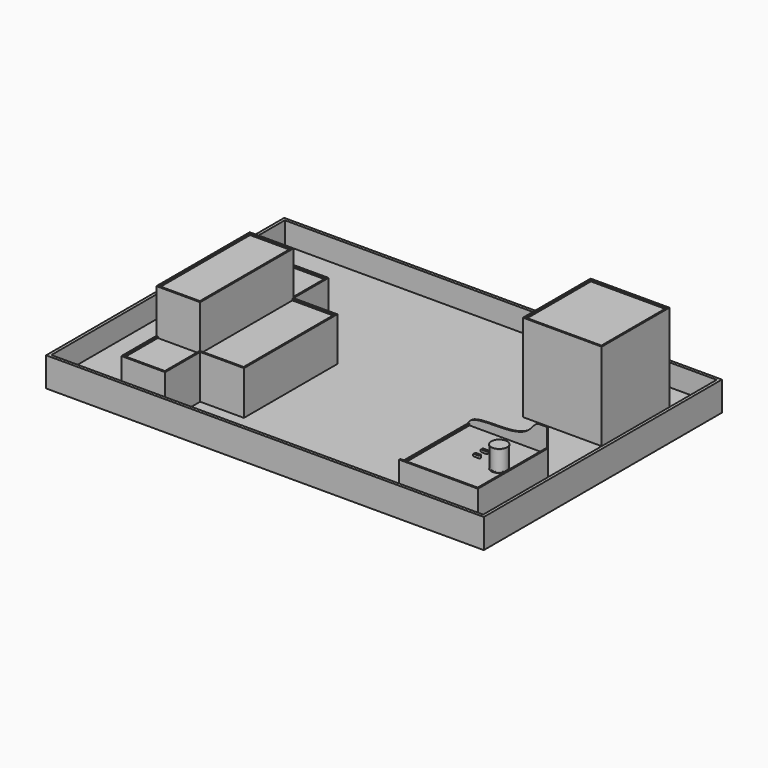
from build123d import *

# Parameters (mm, degrees)
F0_R      = 27.2
F1_DEPTH  = 2.83
F2_R      = 26.4
F3_DEPTH  = 67.36
F4_R      = 27.2
F5_DEPTH  = 2.83
F8_W      = 270
F8_H      = 300
F9_DEPTH  = 72
F11_DEPTH = 15
F13_DEPTH = 5
F14_W     = 5
F14_H     = 290
F15_DEPTH = 5
F16_W     = 1500
F16_H     = 1020
F17_DEPTH = 25
F18_W     = 270
F18_H     = 290
F19_DEPTH = 300
F20_W     = 260
F20_H     = 280
F21_DEPTH = 5
F22_W     = 1500
F22_H     = 1020
F22_W_2   = 1480
F22_H_2   = 1000
F23_DEPTH = 75
F25_DEPTH = 150
F26_W     = 150
F26_H     = 400
F27_DEPTH = 150
F28_W     = 140
F28_H     = 390
F29_DEPTH = 5
F30_W     = 140
F30_H     = 145
F30_W_2   = 145
F30_H_2   = 390
F31_DEPTH = 5
F32_R     = 3
F33_DEPTH = 4
F34_R     = 3.99999
F34_2_R   = 3.99999
F35_R     = 3
F36_DEPTH = 8
F37_R     = 3
F38_DEPTH = 8
F39_R     = 3
F39_R_2   = 2.5
F40_DEPTH = 3
F41_R     = 3
F41_R_2   = 2.5
F42_DEPTH = 3


# Not quite as in the source:
# - a fillet or chamfer is up to 0.001 mm smaller than in the source, because OpenCascade refuses the exact size
# - a feature names something its author has since deleted; it is built from what else it names


with BuildPart() as f1:
    # F0 (on Top) → F1 (new body)
    with BuildSketch(Plane.XY):
        Circle(F0_R)
    extrude(amount=F1_DEPTH)

    # F2 (on face) → F3 (join)
    with BuildSketch(Plane.XY.offset(2.83)):
        Circle(F2_R)
    extrude(amount=F3_DEPTH)

    # F4 (on face) → F5 (join)
    with BuildSketch(Plane.XY.offset(70.19)):
        Circle(F4_R)
    extrude(amount=F5_DEPTH)


with BuildPart() as f9:
    # F8 (on Top) → F9 (new body)
    with BuildSketch(Plane.XY):
        with Locations((-87.8, 0)):
            Rectangle(F8_W, F8_H)
    extrude(amount=-F9_DEPTH)

    # F10 (on face) → F11 (join)
    with BuildSketch(Plane.XY):
        Polygon((-222.8, -145), (-222.8, -150), (47.2, -150), (47.2, 150), (42.2, 150), (42.2, -145), align=None)
    extrude(amount=F11_DEPTH)

    # F12 (on face) → F13 (join)
    with BuildSketch(Plane(origin=(0, 150, 0), x_dir=(-1, 0, 0), z_dir=(0, 1, 0))):
        with BuildLine():
            Line((-21.3134280931, 81.3575685024), (-47.2, 81.3575685024))
            Line((-47.2, 81.3575685024), (-47.2, -72))
            Line((-47.2, -72), (222.8, -72))
            Line((222.8, -72), (222.8, 0))
            add(Edge.make_bspline(
                [(-21.3134280931, 81.3575685024), (-6.3059147253, 81.3822787863), (12.9585432644, 38.1268753575), (103.6097013063, 23.6068887567), (223.0224295336, 30.7718731823), (222.8, 0)],
                knots=[0, 0, 0, 0, 0.2487100673, 0.6151112321, 1, 1, 1, 1], degree=3))
        make_face()
    extrude(amount=-F13_DEPTH)

    # F14 (on face) → F15 (join)
    with BuildSketch(Plane.XY):
        with Locations((-220.3, 0)):
            Rectangle(F14_W, F14_H)
    extrude(amount=F15_DEPTH)

    # F16 (on face) → F17 (join)
    with BuildSketch(Plane(origin=(0, 0, -72), x_dir=(1, 0, 0), z_dir=(0, 0, -1))):
        with Locations((-602.8, -260)):
            Rectangle(F16_W, F16_H)
    extrude(amount=F17_DEPTH)

    # F18 (on face) → F19 (join)
    with BuildSketch(Plane.XY.offset(-72)):
        with Locations((-87.8, 525)):
            Rectangle(F18_W, F18_H)
    extrude(amount=F19_DEPTH)

    # F20 (on face) → F21 (cut)
    with BuildSketch(Plane.XY.offset(228)):
        with Locations((-87.8, 525)):
            Rectangle(F20_W, F20_H)
    extrude(amount=-F21_DEPTH, mode=Mode.SUBTRACT)

    # F22 (on face) → F23 (join)
    with BuildSketch(Plane.XY.offset(-72)):
        with Locations((-602.8, 260)):
            Rectangle(F22_W, F22_H)
        with Locations((-602.8, 260)):
            Rectangle(F22_W_2, F22_H_2, mode=Mode.SUBTRACT)
    extrude(amount=F23_DEPTH)

    # F24 (on face) → F25 (join)
    with BuildSketch(Plane.XY.offset(-72)):
        Polygon((-952.8, 460), (-1102.8, 460), (-1102.8, -240), (-952.8, -240), (-952.8, -90), (-802.8, -90), (-802.8, 310), (-952.8, 310), align=None)
    extrude(amount=F25_DEPTH)

    # F26 (on face) → F27 (join)
    with BuildSketch(Plane.XY.offset(78)):
        with Locations((-1027.8, 110)):
            Rectangle(F26_W, F26_H)
    extrude(amount=F27_DEPTH)

    # F28 (on face) → F29 (cut)
    with BuildSketch(Plane.XY.offset(228)):
        with Locations((-1027.8, 110)):
            Rectangle(F28_W, F28_H)
    extrude(amount=-F29_DEPTH, mode=Mode.SUBTRACT)

    # F30 (on face) → F31 (cut)
    with BuildSketch(Plane.XY.offset(78)):
        with Locations((-1027.8, 382.5)):
            Rectangle(F30_W, F30_H)
        with Locations((-880.3, 110)):
            Rectangle(F30_W_2, F30_H_2)
        with Locations((-1027.8, -162.5)):
            Rectangle(F30_W, F30_H)
    extrude(amount=-F31_DEPTH, mode=Mode.SUBTRACT)


with BuildPart() as f33:
    # F32 (on offset) → F33 (new body, symmetric)
    with BuildSketch(Plane.XY.offset(25)):
        with BuildLine():
            Line((-55, -12), (-74.5, -12))
            Line((-74.5, -12), (-74.5, -13))
            Line((-74.5, -13), (-65.6457513111, -13))
            ThreePointArc((-65.6457513111, -13), (-67, -16), (-65.6457513111, -19))
            Line((-65.6457513111, -19), (-74.5, -19))
            Line((-74.5, -19), (-74.5, -20))
            Line((-74.5, -20), (-55, -20))
            ThreePointArc((-55, -20), (-51, -16), (-55, -12))
        make_face()
        with Locations((-63, -16)):
            Circle(F32_R, mode=Mode.SUBTRACT)
        with Locations((-55, -16)):
            Circle(F32_R, mode=Mode.SUBTRACT)
    extrude(amount=F33_DEPTH, both=True)

    # F34 (radius 4 in the source; OpenCascade refuses exactly that, so slightly less here)
    f34_edges = [f33.edges().sort_by_distance(p)[0] for p in [
        (-74.5, -19.5, 29),
        (-74.5, -12.5, 29),
        (-74.5, -19.5, 21),
        (-74.5, -12.5, 21),
    ]]
    fillet(f34_edges, radius=F34_R)

    # F35 (on face) → F36 (join, through all)
    with BuildSketch(Plane.XZ.offset(20)):
        with Locations((-70.5, 25)):
            Circle(F35_R)
    extrude(amount=-F36_DEPTH)

    # F41 (on offset) → F42 (join, symmetric)
    with BuildSketch(Plane.XY.offset(25)):
        with Locations((-63, -16)):
            Circle(F41_R)
        with Locations((-63, -16)):
            Circle(F41_R_2, mode=Mode.SUBTRACT)
        with Locations((-55, -16)):
            Circle(F41_R)
        with Locations((-55, -16)):
            Circle(F41_R_2, mode=Mode.SUBTRACT)
    extrude(amount=F42_DEPTH, both=True)


with BuildPart() as f33b:
    # F32 (on offset) → F33, piece 2 (new body, symmetric)
    with BuildSketch(Plane.XY.offset(25)):
        with BuildLine():
            Line((-74.5, 13), (-74.5, 12))
            Line((-74.5, 12), (-55, 12))
            ThreePointArc((-55, 12), (-51, 16), (-55, 20))
            Line((-55, 20), (-74.5, 20))
            Line((-74.5, 20), (-74.5, 19))
            Line((-74.5, 19), (-65.6457513111, 19))
            ThreePointArc((-65.6457513111, 19), (-67, 16), (-65.6457513111, 13))
            Line((-65.6457513111, 13), (-74.5, 13))
        make_face()
        with Locations((-63, 16)):
            Circle(F32_R, mode=Mode.SUBTRACT)
        with Locations((-55, 16)):
            Circle(F32_R, mode=Mode.SUBTRACT)
    extrude(amount=F33_DEPTH, both=True)

    # F34#2 (radius 4 in the source; OpenCascade refuses exactly that, so slightly less here)
    f34_2_edges = [f33b.edges().sort_by_distance(p)[0] for p in [
        (-74.5, 12.5, 29),
        (-74.5, 19.5, 29),
        (-74.5, 19.5, 21),
        (-74.5, 12.5, 21),
    ]]
    fillet(f34_2_edges, radius=F34_2_R)

    # F37 (on face) → F38 (join, through all)
    with BuildSketch(Plane(origin=(0, 20, 0), x_dir=(-1, 0, 0), z_dir=(0, 1, 0))):
        with Locations((70.5, 25)):
            Circle(F37_R)
    extrude(amount=-F38_DEPTH)

    # F39 (on offset) → F40 (join, symmetric)
    with BuildSketch(Plane.XY.offset(25)):
        with Locations((-55, 16)):
            Circle(F39_R)
        with Locations((-55, 16)):
            Circle(F39_R_2, mode=Mode.SUBTRACT)
        with Locations((-63, 16)):
            Circle(F39_R)
        with Locations((-63, 16)):
            Circle(F39_R_2, mode=Mode.SUBTRACT)
    extrude(amount=F40_DEPTH, both=True)


solid = Compound([f1.part, f9.part, f33.part, f33b.part])
